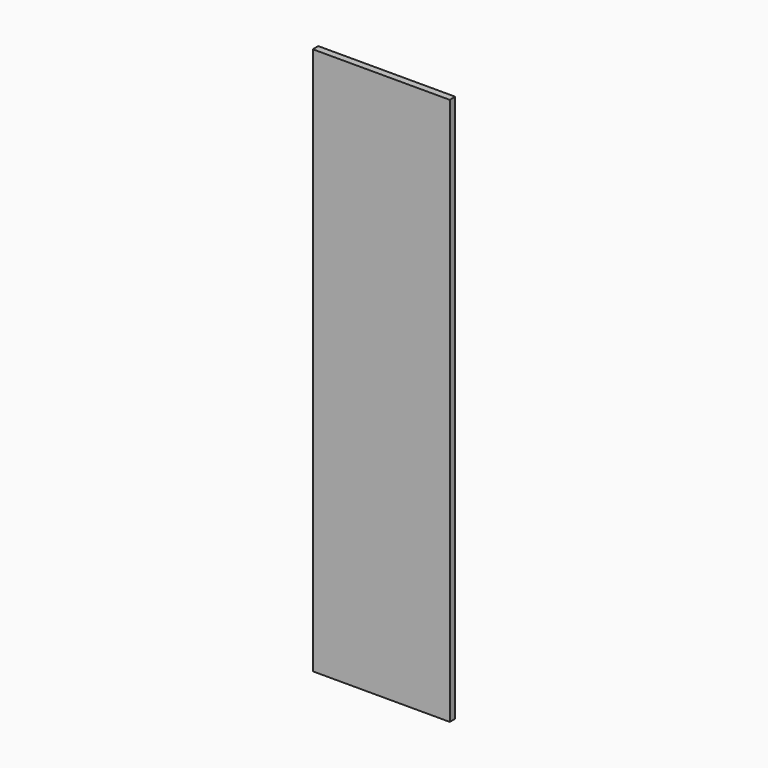
from build123d import *

# Parameters (mm, degrees)
F0_W     = 63.5
F0_H     = 253.87046
F1_DEPTH = 3.175


# Not quite as in the source:
# - a length typed as a fraction of an inch, garbled in the dataset ("3 / 203.2 mm" for 3/8 in), is restored


with BuildPart() as f1:
    # F0 (on Front) → F1 (new body)
    with BuildSketch(Plane.XZ):
        Rectangle(F0_W, F0_H)
    extrude(amount=F1_DEPTH)


solid = f1.part
